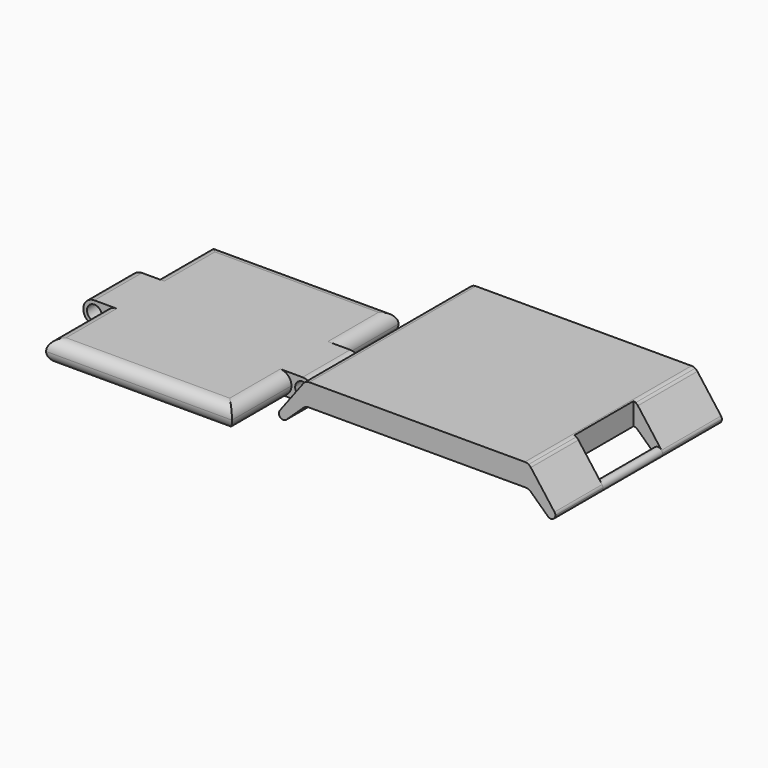
from build123d import *

# Parameters (mm, degrees)
F2_DEPTH  = 28
F3_DEPTH  = 28
F5_DEPTH  = 25
F6_R      = 0.6
F7_DEPTH  = 12
F8_R      = 0.6
F9_DEPTH  = 12
F11_DEPTH = 25
F12_R     = 1.49999


# Not quite as in the source:
# - a fillet or chamfer is up to 0.001 mm smaller than in the source, because OpenCascade refuses the exact size


with BuildPart() as f2:
    # F1 (on face) → F2 (new body)
    with BuildSketch(Plane.XZ):
        with BuildLine():
            Line((-11.068417, 3.007461), (-39.068417, 3.007461))
            Line((-39.068417, 3.007461), (-39.068417, 2.507461))
            ThreePointArc((-39.068417, 2.507461), (-38.36131, 2.214568), (-38.068417, 1.507461))
            ThreePointArc((-38.068417, 1.507461), (-38.36131, 0.800354), (-39.068417, 0.507461))
            Line((-39.068417, 0.507461), (-39.068417, 0.007461))
            Line((-39.068417, 0.007461), (-11.068417, 0.007461))
            Line((-11.068417, 0.007461), (-11.068417, 0.507461))
            ThreePointArc((-11.068417, 0.507461), (-12.068417, 1.507461), (-11.068417, 2.507461))
            Line((-11.068417, 2.507461), (-11.068417, 3.007461))
        make_face()
        with BuildLine():
            Line((-39.068417, 2.507461), (-39.068417, 3.007461))
            ThreePointArc((-39.068417, 3.007461), (-40.568417, 1.507461), (-39.068417, 0.007461))
            Line((-39.068417, 0.007461), (-39.068417, 0.507461))
            ThreePointArc((-39.068417, 0.507461), (-40.068417, 1.507461), (-39.068417, 2.507461))
        make_face()
        with BuildLine():
            ThreePointArc((-11.068417, 0.007461), (-9.568417, 1.507461), (-11.068417, 3.007461))
            Line((-11.068417, 3.007461), (-11.068417, 2.507461))
            ThreePointArc((-11.068417, 2.507461), (-10.36131, 2.214568), (-10.068417, 1.507461))
            ThreePointArc((-10.068417, 1.507461), (-10.36131, 0.800354), (-11.068417, 0.507461))
            Line((-11.068417, 0.507461), (-11.068417, 0.007461))
        make_face()
    extrude(amount=F2_DEPTH)

    # F10 (on face) → F11 (cut)
    with BuildSketch(Plane.XY.offset(3.007461)):
        Polygon((-37.568417, 0), (-39.068417, 0), (-41.568417, 0), (-41.568417, -10), (-37.568417, -10), align=None)
        Polygon((-41.568417, -28), (-39.068417, -28), (-37.568417, -28), (-37.568417, -18), (-41.568417, -18), align=None)
        Polygon((-8.568417, 0), (-11.068417, 0), (-12.568417, 0), (-12.568417, -10), (-8.568417, -10), align=None)
        Polygon((-12.568417, -28), (-11.068417, -28), (-8.568417, -28), (-8.568417, -18), (-12.568417, -18), align=None)
    extrude(amount=-F11_DEPTH, mode=Mode.SUBTRACT)

    # F12 (radius 1.5 in the source; OpenCascade refuses exactly that, so slightly less here)
    f12_edges = [f2.edges().sort_by_distance(p)[0] for p in [
        (-25.068417, -28, 3.007461),
        (-25.068417, 0, 3.007461),
        (-12.568417, -5, 3.007461),
        (-12.568417, -23, 3.007461),
        (-37.568417, -23, 3.007461),
        (-37.568417, -5, 3.007461),
        (-25.068417, 0, 0.007461),
        (-37.568417, -5, 0.007461),
        (-37.568417, -23, 0.007461),
        (-25.068417, -28, 0.007461),
        (-12.568417, -23, 0.007461),
        (-12.568417, -5, 0.007461),
    ]]
    fillet(f12_edges, radius=F12_R)


with BuildPart() as f3:
    # F0 (on Front) → F3 (new body)
    with BuildSketch(Plane.XZ):
        with BuildLine():
            ThreePointArc((-2.95283, 6.100589), (-2.635969, 6.302231), (-2.26707, 6.372762))
            Line((-2.26707, 6.372762), (26.939411, 6.372762))
            ThreePointArc((26.939411, 6.372762), (27.308098, 6.302316), (27.624839, 6.100903))
            Line((27.624839, 6.100903), (29.924782, 3.935877))
            ThreePointArc((29.924782, 3.935877), (29.936116, 4.820045), (30.816038, 4.732762))
            Line((30.816038, 4.732762), (27.636038, 8.972762))
            ThreePointArc((27.636038, 8.972762), (27.499508, 9.120965), (27.336038, 9.238787))
            ThreePointArc((27.336038, 9.238787), (27.094857, 9.338688), (26.836038, 9.372762))
            Line((26.836038, 9.372762), (-2.163817, 9.372762))
            ThreePointArc((-2.163817, 9.372762), (-2.422717, 9.338666), (-2.663962, 9.238704))
            ThreePointArc((-2.663962, 9.238704), (-2.827436, 9.120833), (-2.963956, 8.972577))
            Line((-2.963956, 8.972577), (-6.144045, 4.730413))
            ThreePointArc((-6.144045, 4.730413), (-5.474291, 4.939756), (-5.063962, 4.370525))
            ThreePointArc((-5.063962, 4.370525), (-5.113111, 4.132695), (-5.252505, 3.933828))
            Line((-5.252505, 3.933828), (-2.95283, 6.100589))
        make_face()
        with BuildLine():
            ThreePointArc((-6.144045, 4.730413), (-6.06373, 3.923103), (-5.252505, 3.933828))
            ThreePointArc((-5.252505, 3.933828), (-5.113111, 4.132695), (-5.063962, 4.370525))
            ThreePointArc((-5.063962, 4.370525), (-5.474291, 4.939756), (-6.144045, 4.730413))
        make_face()
        with BuildLine():
            ThreePointArc((30.816038, 4.732762), (29.936116, 4.820045), (29.924782, 3.935877))
            ThreePointArc((29.924782, 3.935877), (30.573994, 3.821965), (30.936038, 4.372762))
            ThreePointArc((30.936038, 4.372762), (30.905248, 4.562499), (30.816038, 4.732762))
        make_face()
    extrude(amount=F3_DEPTH)

    # F4 (on face) → F5 (cut)
    with BuildSketch(Plane.XY.offset(9.372762)):
        Polygon((27.068583, -10), (27.068583, -15), (27.068583, -20), (31.068583, -20), (31.068583, -10), align=None)
        Polygon((-2.931417, -20), (-2.931417, -15), (-2.931417, -10), (-6.931417, -10), (-6.931417, -20), align=None)
    extrude(amount=-F5_DEPTH, mode=Mode.SUBTRACT)

    # F6 (on face) → F7 (join)
    with BuildSketch(Plane.XZ.offset(10)):
        with Locations((30.336038, 4.372762)):
            Circle(F6_R)
    extrude(amount=F7_DEPTH)

    # F8 (on face) → F9 (join)
    with BuildSketch(Plane.XZ.offset(10)):
        with Locations((-5.663962, 4.370525)):
            Circle(F8_R)
    extrude(amount=F9_DEPTH)


solid = Compound([f2.part, f3.part])
